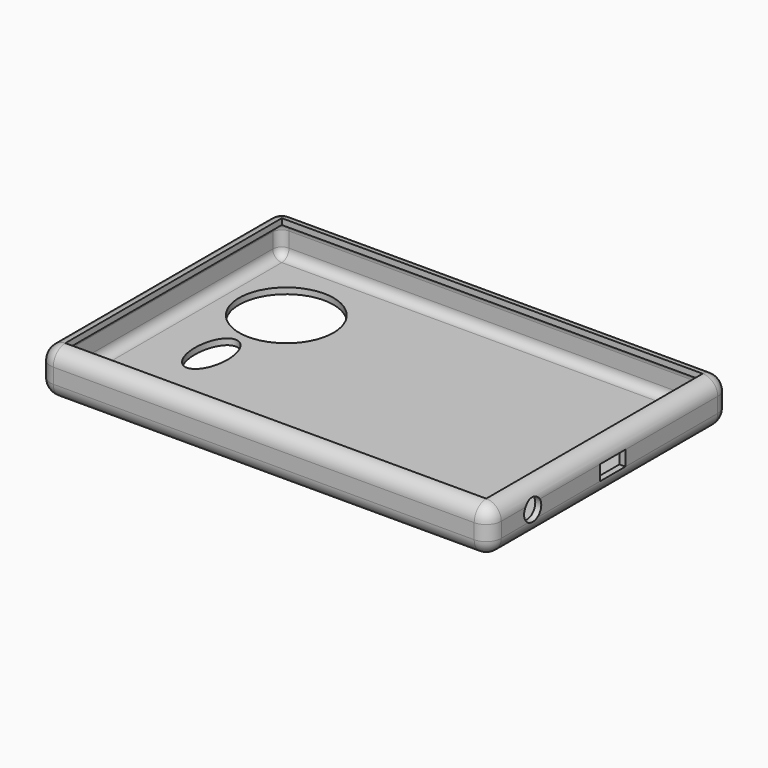
from build123d import *

# Parameters (mm, degrees)
F0_W         = 150
F0_H         = 100
F1_DEPTH     = 15
F2_R         = 5
F3_T1_DEPTH  = 5
F3_S5_W      = 5
F3_S5_H      = 5
F3_T6_DEPTH  = 5
F3_S11_W     = 5
F3_S11_H     = 5
F3_T12_DEPTH = 5
F4_T         = -2
F6_R         = 15.7014328103
F7_DEPTH     = 25
F8_W         = 10.624602437
F8_H         = 5
F8_R         = 3.5673659444
F9_DEPTH     = 25


# Not quite as in the source:
# - a fillet or chamfer that OpenCascade refuses, or shapes differently, is made with other operations: its cross-section is extruded or revolved along the edge and cut away or added
# - a shell that OpenCascade refuses in one call is made with other operations: the cavity is built on its own and cut out


with BuildPart() as f1:
    # F0 (on Top) → F1 (new body)
    with BuildSketch(Plane.XY):
        Rectangle(F0_W, F0_H)
    extrude(amount=F1_DEPTH)

    # F2
    f2_edges = [f1.edges().sort_by_distance(p)[0] for p in [
        (-75, 50, 7.5),
        (-75, -50, 7.5),
        (75, -50, 7.5),
        (0, 50, 0),
        (0, -50, 0),
        (0, -50, 15),
        (-75, 0, 0),
        (-75, 0, 15),
        (75, 0, 0),
        (0, 50, 15),
        (75, 0, 15),
    ]]
    fillet(f2_edges, radius=F2_R)

    # F3: fillet of radius 5 on 1 edges, made by hand

    # F3_s2 → F3_t1 (cut)
    with BuildSketch(Plane.XY.offset(5)):
        with BuildLine():
            ThreePointArc((70, 50), (73.5355339059, 48.5355339059), (75, 45))
            Line((75, 45), (75, 50))
            Line((75, 50), (70, 50))
        make_face()
    extrude(amount=F3_T1_DEPTH, mode=Mode.SUBTRACT)


with BuildPart() as f3_tool4:
    # F3_s5 → F3_t6 (new body)
    with BuildSketch(Plane.XZ.offset(-45)):
        with Locations((72.5, 2.5)):
            Rectangle(F3_S5_W, F3_S5_H)
    extrude(amount=-F3_T6_DEPTH)

    # F3_s7 → F3_t8 (revolve, cut)
    with BuildSketch(Plane(origin=(70, 45, 5), x_dir=(-0.7071067812, 0, 0.7071067812), z_dir=(-0.7071067812, 0, -0.7071067812))):
        with BuildLine():
            ThreePointArc((0, -5), (5, 0), (0, 5))
            Line((0, 5), (0, -5))
        make_face()
    revolve(axis=Axis((70, 45, 5), (0, 1, 0)), mode=Mode.SUBTRACT)


with BuildPart() as f1_1:
    add(f1.part)

    # F3_t3: cut F3_tool4
    add(f3_tool4.part, mode=Mode.SUBTRACT)


with BuildPart() as f3_tool10:
    # F3_s11 → F3_t12 (new body)
    with BuildSketch(Plane.XZ.offset(-45)):
        with Locations((72.5, 12.5)):
            Rectangle(F3_S11_W, F3_S11_H)
    extrude(amount=-F3_T12_DEPTH)

    # F3_s13 → F3_t14 (revolve, cut)
    with BuildSketch(Plane(origin=(70, 45, 10), x_dir=(-0.7071067812, 0, -0.7071067812), z_dir=(0.7071067812, 0, -0.7071067812))):
        with BuildLine():
            ThreePointArc((0, -5), (5, 0), (0, 5))
            Line((0, 5), (0, -5))
        make_face()
    revolve(axis=Axis((70, 45, 10), (0, 1, 0)), mode=Mode.SUBTRACT)


with BuildPart() as f1_2:
    add(f1_1.part)

    # F3_t9: cut F3_tool10
    add(f3_tool10.part, mode=Mode.SUBTRACT)

    # F4: a shell. OpenCascade refuses it in one call, so the cavity is built on its own and cut out:
    # the body offset inwards by the wall thickness, plus a prism from it out through each open face.
    f4_core = offset(f1_2.part, amount=F4_T, mode=Mode.PRIVATE)
    f4_exits = [f4_core.faces().sort_by_distance(p)[0] for p in [
        (0, 0, 13),
    ]]
    add(f4_core, mode=Mode.SUBTRACT)
    extrude(f4_exits, amount=-F4_T, mode=Mode.SUBTRACT)

    # F6 (on face) → F7 (cut)
    with BuildSketch(Plane(origin=(0, 0, 0), x_dir=(1, 0, 0), z_dir=(0, 0, -1))):
        with Locations((-50.5510754883, -22.5712861866)):
            Circle(F6_R)
        with BuildLine():
            add(Edge.make_bspline(
                [(-52.28683725, 16.5926627815), (-61.667239248, 16.5926627815), (-56.977038249, 1.3871968258), (-52.28683725, -13.8182691298), (-47.596636251, 1.3871968258), (-42.906435252, 16.5926627815), (-52.28683725, 16.5926627815)],
                knots=[0, 0, 0, 2.0943951024, 2.0943951024, 4.1887902048, 4.1887902048, 6.2831853072, 6.2831853072, 6.2831853072], degree=2, weights=[1, 0.5, 1, 0.5, 1, 0.5, 1]))
        make_face()
    extrude(amount=-F7_DEPTH, mode=Mode.SUBTRACT)

    # F8 (on face) → F9 (cut)
    with BuildSketch(Plane.YZ.offset(75)):
        with Locations((1.3190158643, 7.5)):
            Rectangle(F8_W, F8_H)
        with Locations((-31.9286696613, 8.0319177359)):
            Circle(F8_R)
    extrude(amount=-F9_DEPTH, mode=Mode.SUBTRACT)


solid = f1_2.part
